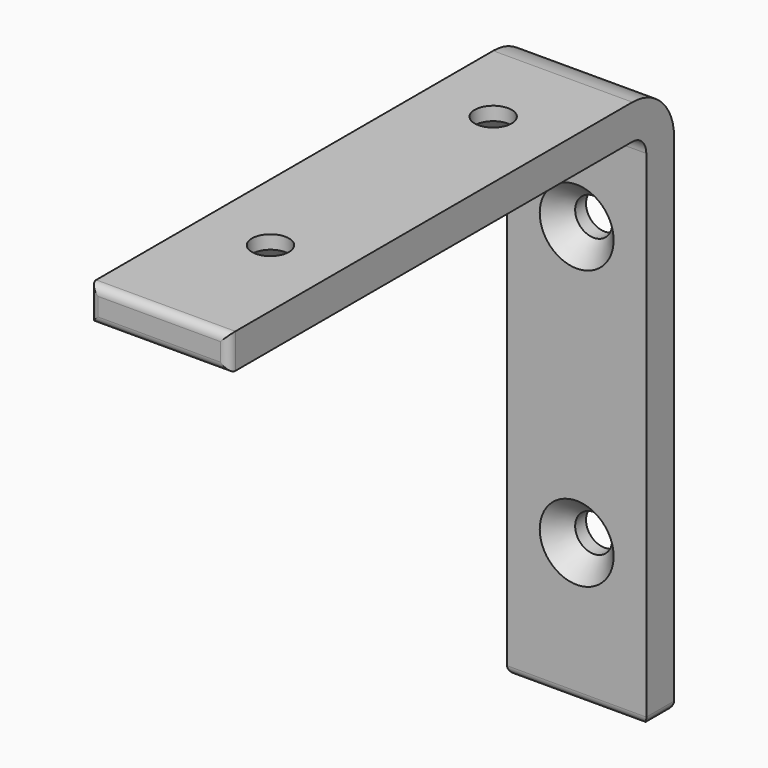
from build123d import *

# Parameters (mm, degrees)
F1_DEPTH       = 12.7
F3_D           = 6.7564
F3_CSINK_D     = 13.4874
F3_CSINK_ANGLE = 82
F5_D           = 6.7564
F5_CSINK_D     = 13.4874
F5_CSINK_ANGLE = 82
F6_R           = 3.175
F7_R           = 9.525
F8_R           = 1.524


with BuildPart() as f1:
    # F0 (on Right) → F1 (new body, symmetric)
    with BuildSketch(Plane.YZ):
        Polygon((-36.0811725259, 16.0017143935), (-36.0811725259, 9.6517140046), (59.1688280165, 9.6517140046), (59.1688280165, -85.5982856065), (65.5188274741, -85.5982856065), (65.5188274741, 16.0017143935), align=None)
    extrude(amount=F1_DEPTH, both=True)

    # F3 (through all)
    with Locations(Plane.XZ.offset(-59.1688280165)):
        with Locations((0, -9.3982859954), (0, -60.1982859954)):
            CounterSinkHole(F3_D / 2, F3_CSINK_D / 2, counter_sink_angle=F3_CSINK_ANGLE)

    # F5 (through all)
    with Locations(Plane(origin=(0, 0, 9.6517140046), x_dir=(1, 0, 0), z_dir=(0, 0, -1))):
        with Locations((0, 10.6811719835), (0, -40.1188280165)):
            CounterSinkHole(F5_D / 2, F5_CSINK_D / 2, counter_sink_angle=F5_CSINK_ANGLE)

    # F6
    f6_edges = [f1.edges().sort_by_distance(p)[0] for p in [
        (0, 59.168828, 9.651714),
    ]]
    fillet(f6_edges, radius=F6_R)

    # F7
    f7_edges = [f1.edges().sort_by_distance(p)[0] for p in [
        (0, 65.518827, 16.001714),
    ]]
    fillet(f7_edges, radius=F7_R)

    # F8
    f8_edges = [f1.edges().sort_by_distance(p)[0] for p in [
        (12.7, 62.343828, -85.598286),
        (12.7, -36.081173, 12.826714),
        (-12.7, -36.081173, 12.826714),
        (-12.7, 62.343828, -85.598286),
        (0, 65.518827, -85.598286),
        (0, -36.081173, 16.001714),
        (0, -36.081173, 9.651714),
        (0, 59.168828, -85.598286),
    ]]
    fillet(f8_edges, radius=F8_R)


solid = f1.part
